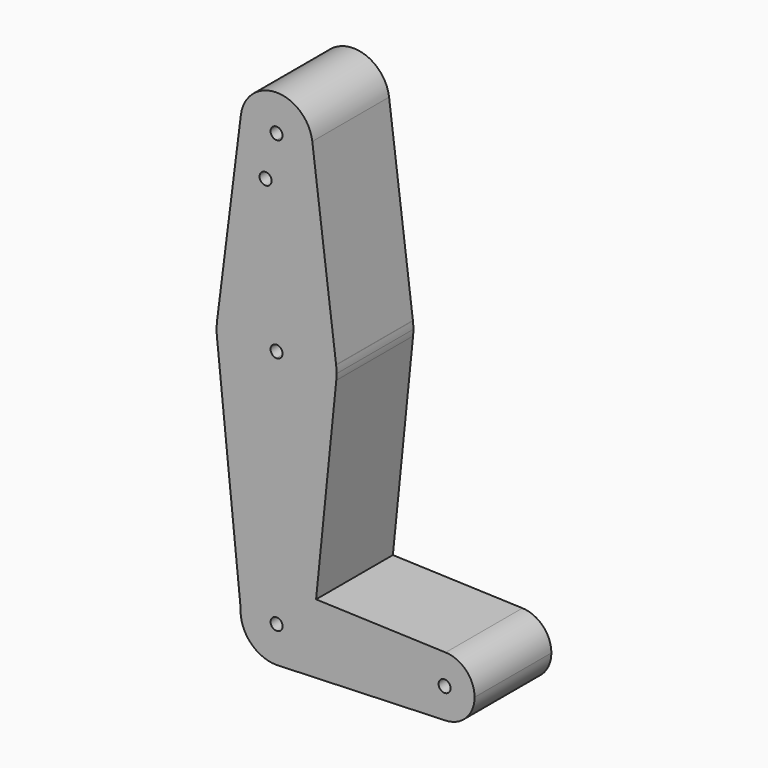
from build123d import *

# Parameters (mm, degrees)
F0_R     = 1.5875
F1_DEPTH = 25.4


# Not quite as in the source:
# - ends of sketch curves that miss each other by under 0.0002 mm in the source are joined


with BuildPart() as f1:
    # F0 (on Front) → F1 (new body)
    with BuildSketch(Plane.XZ):
        with BuildLine():
            ThreePointArc((1.5875, 0), (-1.1225320151, -1.1225320151), (0, 1.5875))
            Line((0, 1.5875), (0, 9.525))
            ThreePointArc((0, 9.525), (-6.5322234356, 6.9322205668), (-9.5082023407, 0.5654319132))
            ThreePointArc((-9.5082023407, 0.5654319132), (-6.9322205668, -6.5322234356), (0, -9.525))
            Line((0, -9.525), (0.6773435479, -9.500885786))
            ThreePointArc((0.6773435479, -9.500885786), (6.9705567315, -6.4912990883), (9.525, 0))
            Line((9.525, 0), (1.5875, 0))
        make_face()
        with BuildLine():
            ThreePointArc((-9.5082023407, 0.5654319132), (-6.5322234356, 6.9322205668), (0, 9.525))
            Line((0, 9.525), (0, 47.625))
            ThreePointArc((0, 47.625), (-10.5003255158, 51.59375), (-15.7504882737, 61.515625))
            Line((-15.7504882737, 61.515625), (-9.5082023407, 0.5654319132))
        make_face()
        with BuildLine():
            Line((0, 47.625), (0, 9.525))
            ThreePointArc((0, 9.525), (0.3388863295, 9.5189695375), (0.6773435479, 9.500885786))
            Line((0.6773435479, 9.500885786), (10.4519953809, 9.152896871))
            Line((10.4519953809, 9.152896871), (15.7942028036, 61.9003804205))
            ThreePointArc((15.7942028036, 61.9003804205), (10.644756084, 51.722700101), (0, 47.625))
        make_face()
        with BuildLine():
            Line((10.4519953809, 9.152896871), (9.525, 0))
            Line((9.525, 0), (36.5125, 0))
            ThreePointArc((36.5125, 0), (38.9380895153, 5.7116327839), (44.7324052746, 7.9324746146))
            Line((44.7324052746, 7.9324746146), (10.4519953809, 9.152896871))
        make_face()
        with BuildLine():
            Line((36.5125, 0), (9.525, 0))
            ThreePointArc((9.525, 0), (6.9705567315, -6.4912990883), (0.6773435479, -9.500885786))
            Line((0.6773435479, -9.500885786), (44.7324052746, -7.9324746146))
            ThreePointArc((44.7324052746, -7.9324746146), (38.9380895153, -5.7116327839), (36.5125, 0))
        make_face()
        with BuildLine():
            ThreePointArc((0.6773435479, 9.500885786), (6.9705567315, 6.4912990883), (9.525, 0))
            Line((9.525, 0), (10.4519953809, 9.152896871))
            Line((10.4519953809, 9.152896871), (0.6773435479, 9.500885786))
        make_face()
        with BuildLine():
            ThreePointArc((-15.7504882737, 61.515625), (-10.5003255158, 51.59375), (0, 47.625))
            Line((0, 47.625), (0, 61.9125))
            ThreePointArc((0, 61.9125), (-1.5875, 63.5), (0, 65.0875))
            Line((0, 65.0875), (0, 79.375))
            ThreePointArc((0, 79.375), (-10.5003255158, 75.40625), (-15.7504882737, 65.484375))
            ThreePointArc((-15.7504882737, 65.484375), (-15.875, 63.5), (-15.7504882737, 61.515625))
        make_face()
        with BuildLine():
            ThreePointArc((0, 79.375), (10.5154665352, 75.3928797415), (15.7554871092, 65.444286746))
            Line((15.7554871092, 65.444286746), (9.4502929642, 115.490625))
            ThreePointArc((9.4502929642, 115.490625), (9.5063048942, 114.896483242), (9.525, 114.3))
            ThreePointArc((9.525, 114.3), (6.7351920908, 107.5648079092), (0, 104.775))
            Line((0, 104.775), (0, 79.375))
        make_face()
        with BuildLine():
            Line((0, 61.9125), (0, 47.625))
            ThreePointArc((0, 47.625), (10.644756084, 51.722700101), (15.7942028036, 61.9003804205))
            ThreePointArc((15.7942028036, 61.9003804205), (15.8547878338, 62.6991705884), (15.875, 63.5))
            ThreePointArc((15.875, 63.5), (15.8450936075, 64.4739782187), (15.7554871092, 65.444286746))
            ThreePointArc((15.7554871092, 65.444286746), (10.5154665352, 75.3928797415), (0, 79.375))
            Line((0, 79.375), (0, 65.0875))
            ThreePointArc((0, 65.0875), (1.1225320151, 64.6225320151), (1.5875, 63.5))
            ThreePointArc((1.5875, 63.5), (1.1225320151, 62.3774679849), (0, 61.9125))
        make_face()
        with BuildLine():
            ThreePointArc((44.7324052746, 7.9324746146), (38.9380895153, 5.7116327839), (36.5125, 0))
            ThreePointArc((36.5125, 0), (38.9380895153, -5.7116327839), (44.7324052746, -7.9324746146))
            ThreePointArc((44.7324052746, -7.9324746146), (50.1616327839, -5.5119104847), (52.3875, 0))
            ThreePointArc((52.3875, 0), (50.1616327839, 5.5119104847), (44.7324052746, 7.9324746146))
        make_face()
        with BuildLine():
            ThreePointArc((46.0375, 0), (44.45, -1.5875), (42.8625, 0))
            ThreePointArc((42.8625, 0), (44.45, 1.5875), (46.0375, 0))
        make_face(mode=Mode.SUBTRACT)
        with BuildLine():
            ThreePointArc((0, -9.525), (0.3388863295, -9.5189695375), (0.6773435479, -9.500885786))
            Line((0.6773435479, -9.500885786), (0, -9.525))
        make_face()
        with BuildLine():
            Line((-9.4502929642, 115.490625), (-15.7504882737, 65.484375))
            ThreePointArc((-15.7504882737, 65.484375), (-10.5003255158, 75.40625), (0, 79.375))
            Line((0, 79.375), (0, 104.775))
            ThreePointArc((0, 104.775), (-7.14375, 107.9998046905), (-9.4502929642, 115.490625))
        make_face()
        with Locations((-2.919731196, 102.79443115)):
            Circle(F0_R, mode=Mode.SUBTRACT)
        with BuildLine():
            ThreePointArc((9.4502929642, 115.490625), (0, 123.825), (-9.4502929642, 115.490625))
            ThreePointArc((-9.4502929642, 115.490625), (-7.14375, 107.9998046905), (0, 104.775))
            ThreePointArc((0, 104.775), (6.7351920908, 107.5648079092), (9.525, 114.3))
            ThreePointArc((9.525, 114.3), (9.5063048942, 114.896483242), (9.4502929642, 115.490625))
        make_face()
        with BuildLine():
            ThreePointArc((1.5875, 114.3), (1.1225320151, 113.1774679849), (0, 112.7125))
            ThreePointArc((0, 112.7125), (-1.1225320151, 115.4225320151), (1.5875, 114.3))
        make_face(mode=Mode.SUBTRACT)
        with BuildLine():
            Line((0, 9.525), (0, 1.5875))
            ThreePointArc((0, 1.5875), (1.1225320151, 1.1225320151), (1.5875, 0))
            Line((1.5875, 0), (9.525, 0))
            ThreePointArc((9.525, 0), (6.9705567315, 6.4912990883), (0.6773435479, 9.500885786))
            Line((0.6773435479, 9.500885786), (0, 9.525))
        make_face()
    extrude(amount=F1_DEPTH)


solid = f1.part
